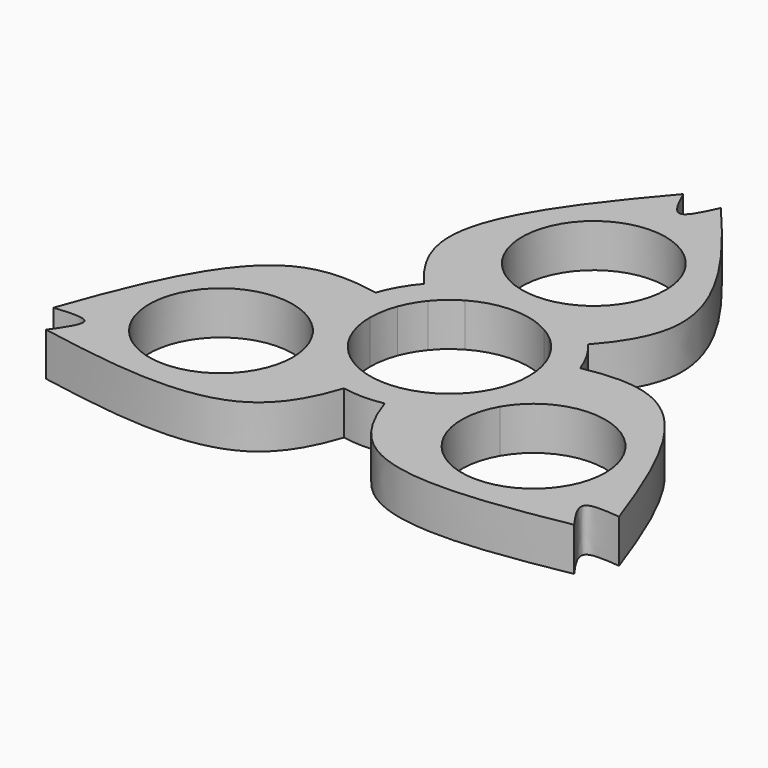
from build123d import *

# Parameters (mm, degrees)
F0_R     = 9.95
F1_DEPTH = 6


with BuildPart() as f1:
    # F0 (on Top) → F1 (new body)
    with BuildSketch(Plane.XY):
        with BuildLine():
            ThreePointArc((5.5, 9.5262794416), (6.3093407999, 9.0106724872), (7.0706637066, 8.4264888743))
            ThreePointArc((7.0706637066, 8.4264888743), (7.8268557987, 7.7291867817), (8.5146077493, 6.9642985918))
            add(Edge.make_bspline(
                [(8.5146077493, 6.9642985918), (9.5301249028, 7.9008868503), (10.4822945034, 8.8485192108), (11.3460669028, 9.8115628642)],
                knots=[0.1806363612, 0.1806363612, 0.1806363612, 0.1806363612, 0.2520657546, 0.2520657546, 0.2520657546, 0.2520657546], degree=3))
            add(Edge.make_bspline(
                [(11.3460669028, 9.8115628642), (13.9736725709, 12.7411528396), (19.7429640918, 22.5358646022), (10.0301146668, 35.0297546933), (2.6054169788, 43.7370347171)],
                knots=[0.2520657546, 0.2520657546, 0.2520657546, 0.2520657546, 0.4693547987, 0.9448204936, 0.9448204936, 0.9448204936, 0.9448204936], degree=3))
            add(Edge.make_bspline(
                [(-2.6054169788, 43.7370347171), (-1.7369446525, 41.8435173586), (0, 38.0564826414), (1.7369446525, 41.8435173586), (2.6054169788, 43.7370347171)],
                knots=[0, 0, 0, 0, 0.5, 1, 1, 1, 1], degree=3))
            add(Edge.make_bspline(
                [(-11.3460669028, 9.8115628642), (-13.9736725709, 12.7411528396), (-19.7429640918, 22.5358646022), (-10.0301146668, 35.0297546933), (-2.6054169788, 43.7370347171)],
                knots=[0.2520657546, 0.2520657546, 0.2520657546, 0.2520657546, 0.4693547987, 0.9448204936, 0.9448204936, 0.9448204936, 0.9448204936], degree=3))
            add(Edge.make_bspline(
                [(-8.5146077493, 6.9642985918), (-9.5301249028, 7.9008868503), (-10.4822945034, 8.8485192108), (-11.3460669028, 9.8115628642)],
                knots=[0.1806363612, 0.1806363612, 0.1806363612, 0.1806363612, 0.2520657546, 0.2520657546, 0.2520657546, 0.2520657546], degree=3))
            ThreePointArc((-8.5146077493, 6.9642985918), (-7.1234292346, 8.381930323), (-5.5, 9.5262794416))
            ThreePointArc((-5.5, 9.5262794416), (0, 11), (5.5, 9.5262794416))
        make_face()
        with BuildLine():
            ThreePointArc((0, 15.05), (-7.0357124728, 32.0357124728), (9.95, 25))
            ThreePointArc((9.95, 25), (7.0357124728, 17.9642875272), (0, 15.05))
        make_face(mode=Mode.SUBTRACT)
        with BuildLine():
            add(Edge.make_bspline(
                [(8.5146077493, 6.9642985918), (9.5301249028, 7.9008868503), (10.4822945034, 8.8485192108), (11.3460669028, 9.8115628642)],
                knots=[0.1806363612, 0.1806363612, 0.1806363612, 0.1806363612, 0.2520657546, 0.2520657546, 0.2520657546, 0.2520657546], degree=3))
            ThreePointArc((8.5146077493, 6.9642985918), (9.5262794416, 5.5), (10.2885633747, 3.8917173182))
            add(Edge.make_bspline(
                [(10.2885633747, 3.8917173182), (11.6074311762, 4.3028868419), (12.9041896741, 4.6536737245), (14.1700961426, 4.9202007387)],
                knots=[0.1806363612, 0.1806363612, 0.1806363612, 0.1806363612, 0.2520657546, 0.2520657546, 0.2520657546, 0.2520657546], degree=3))
            ThreePointArc((14.1700961426, 4.9202007387), (12.9903810568, 7.5), (11.3460669028, 9.8115628642))
        make_face()
        with BuildLine():
            add(Edge.make_bspline(
                [(10.2885633747, 3.8917173182), (11.6074311762, 4.3028868419), (12.9041896741, 4.6536737245), (14.1700961426, 4.9202007387)],
                knots=[0.1806363612, 0.1806363612, 0.1806363612, 0.1806363612, 0.2520657546, 0.2520657546, 0.2520657546, 0.2520657546], degree=3))
            ThreePointArc((10.2885633747, 3.8917173182), (10.8206792098, 1.9781055177), (11, 0))
            ThreePointArc((11, 0), (9.5262794416, -5.5), (5.5, -9.5262794416))
            ThreePointArc((5.5, -9.5262794416), (3.6972499752, -10.3600358407), (1.7739556254, -10.85601591))
            add(Edge.make_bspline(
                [(1.7739556254, -10.85601591), (2.0773062734, -12.2037736923), (2.4218951707, -13.5021929353), (2.8240292398, -14.7317636029)],
                knots=[0.1806363612, 0.1806363612, 0.1806363612, 0.1806363612, 0.2520657546, 0.2520657546, 0.2520657546, 0.2520657546], degree=3))
            add(Edge.make_bspline(
                [(2.8240292398, -14.7317636029), (4.0473257472, -18.4721318504), (9.6451491958, -28.3658407506), (25.3216001194, -26.201211451), (36.5746746618, -24.1248746496)],
                knots=[0.2520657546, 0.2520657546, 0.2520657546, 0.2520657546, 0.4693547987, 0.9448204936, 0.9448204936, 0.9448204936, 0.9448204936], degree=3))
            add(Edge.make_bspline(
                [(36.5746746618, -24.1248746496), (35.3690766899, -22.4259968733), (32.9578807462, -19.0282413207), (37.1060213425, -19.4175204852), (39.1800916406, -19.6121600675)],
                knots=[0, 0, 0, 0, 0.5, 1, 1, 1, 1], degree=3))
            add(Edge.make_bspline(
                [(14.1700961426, 4.9202007387), (18.0209983181, 5.7309790107), (29.3881132876, 5.8299761484), (35.3517147861, -8.8285432423), (39.1800916406, -19.6121600675)],
                knots=[0.2520657546, 0.2520657546, 0.2520657546, 0.2520657546, 0.4693547987, 0.9448204936, 0.9448204936, 0.9448204936, 0.9448204936], degree=3))
        make_face()
        with BuildLine():
            ThreePointArc((13.033682327, -7.525), (24.2258845934, -2.8890380284), (31.6006350946, -12.5))
            ThreePointArc((31.6006350946, -12.5), (19.0753855958, -22.1109619716), (13.033682327, -7.525))
        make_face(mode=Mode.SUBTRACT)
        with BuildLine():
            ThreePointArc((-10.2885633747, 3.8917173182), (-9.5262794416, 5.5), (-8.5146077493, 6.9642985918))
            add(Edge.make_bspline(
                [(-8.5146077493, 6.9642985918), (-9.5301249028, 7.9008868503), (-10.4822945034, 8.8485192108), (-11.3460669028, 9.8115628642)],
                knots=[0.1806363612, 0.1806363612, 0.1806363612, 0.1806363612, 0.2520657546, 0.2520657546, 0.2520657546, 0.2520657546], degree=3))
            ThreePointArc((-11.3460669028, 9.8115628642), (-12.9903810568, 7.5), (-14.1700961426, 4.9202007387))
            add(Edge.make_bspline(
                [(-10.2885633747, 3.8917173182), (-11.6074311762, 4.3028868419), (-12.9041896741, 4.6536737245), (-14.1700961426, 4.9202007387)],
                knots=[0.1806363612, 0.1806363612, 0.1806363612, 0.1806363612, 0.2520657546, 0.2520657546, 0.2520657546, 0.2520657546], degree=3))
        make_face()
        with BuildLine():
            add(Edge.make_bspline(
                [(1.7739556254, -10.85601591), (2.0773062734, -12.2037736923), (2.4218951707, -13.5021929353), (2.8240292398, -14.7317636029)],
                knots=[0.1806363612, 0.1806363612, 0.1806363612, 0.1806363612, 0.2520657546, 0.2520657546, 0.2520657546, 0.2520657546], degree=3))
            ThreePointArc((1.7739556254, -10.85601591), (0, -11), (-1.7739556254, -10.85601591))
            add(Edge.make_bspline(
                [(-1.7739556254, -10.85601591), (-2.0773062734, -12.2037736923), (-2.4218951707, -13.5021929353), (-2.8240292398, -14.7317636029)],
                knots=[0.1806363612, 0.1806363612, 0.1806363612, 0.1806363612, 0.2520657546, 0.2520657546, 0.2520657546, 0.2520657546], degree=3))
            ThreePointArc((-2.8240292398, -14.7317636029), (0, -15), (2.8240292398, -14.7317636029))
        make_face()
        with BuildLine():
            ThreePointArc((-11, 0), (-10.8206792098, 1.9781055177), (-10.2885633747, 3.8917173182))
            add(Edge.make_bspline(
                [(-10.2885633747, 3.8917173182), (-11.6074311762, 4.3028868419), (-12.9041896741, 4.6536737245), (-14.1700961426, 4.9202007387)],
                knots=[0.1806363612, 0.1806363612, 0.1806363612, 0.1806363612, 0.2520657546, 0.2520657546, 0.2520657546, 0.2520657546], degree=3))
            add(Edge.make_bspline(
                [(-14.1700961426, 4.9202007387), (-18.0209983181, 5.7309790107), (-29.3881132876, 5.8299761484), (-35.3517147861, -8.8285432423), (-39.1800916406, -19.6121600675)],
                knots=[0.2520657546, 0.2520657546, 0.2520657546, 0.2520657546, 0.4693547987, 0.9448204936, 0.9448204936, 0.9448204936, 0.9448204936], degree=3))
            add(Edge.make_bspline(
                [(-39.1800916406, -19.6121600675), (-37.1060213425, -19.4175204852), (-32.9578807462, -19.0282413207), (-35.3690766899, -22.4259968733), (-36.5746746618, -24.1248746496)],
                knots=[0, 0, 0, 0, 0.5, 1, 1, 1, 1], degree=3))
            add(Edge.make_bspline(
                [(-2.8240292398, -14.7317636029), (-4.0473257472, -18.4721318504), (-9.6451491958, -28.3658407506), (-25.3216001194, -26.201211451), (-36.5746746618, -24.1248746496)],
                knots=[0.2520657546, 0.2520657546, 0.2520657546, 0.2520657546, 0.4693547987, 0.9448204936, 0.9448204936, 0.9448204936, 0.9448204936], degree=3))
            add(Edge.make_bspline(
                [(-1.7739556254, -10.85601591), (-2.0773062734, -12.2037736923), (-2.4218951707, -13.5021929353), (-2.8240292398, -14.7317636029)],
                knots=[0.1806363612, 0.1806363612, 0.1806363612, 0.1806363612, 0.2520657546, 0.2520657546, 0.2520657546, 0.2520657546], degree=3))
            ThreePointArc((-1.7739556254, -10.85601591), (-3.6972499752, -10.3600358407), (-5.5, -9.5262794416))
            ThreePointArc((-5.5, -9.5262794416), (-9.5262794416, -5.5), (-11, 0))
        make_face()
        with Locations((-21.6506350946, -12.5)):
            Circle(F0_R, mode=Mode.SUBTRACT)
    extrude(amount=F1_DEPTH)


solid = f1.part
